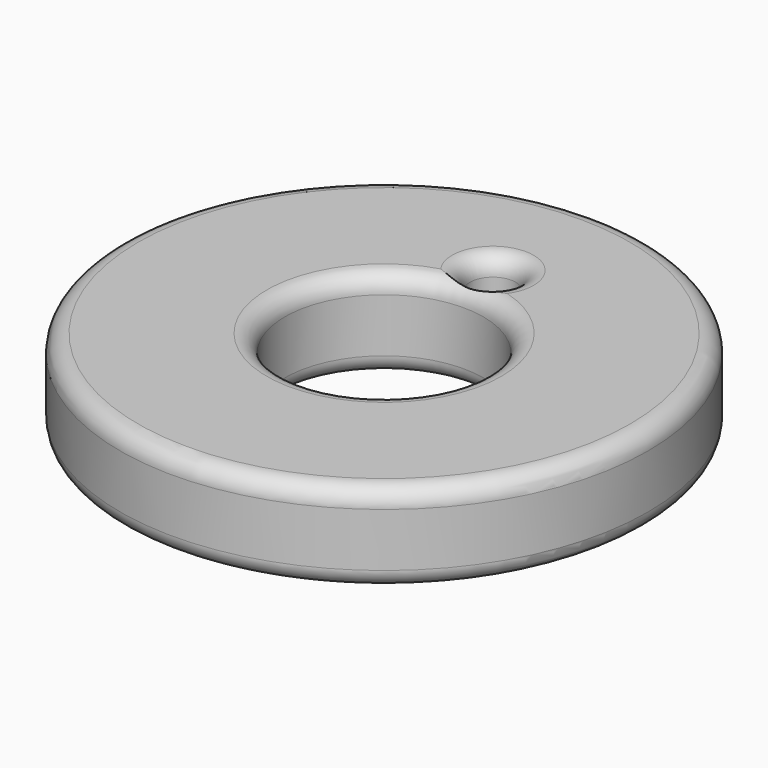
from build123d import *

# Parameters (mm, degrees)
F0_R     = 74.892271749
F0_R_2   = 28.179048931
F0_R_3   = 6.4977417518
F1_DEPTH = 25.4


# Not quite as in the source:
# - a fillet or chamfer that OpenCascade refuses, or shapes differently, is made with other operations: its cross-section is extruded or revolved along the edge and cut away or added


with BuildPart() as f1:
    # F0 (on Top) → F1 (new body)
    with BuildSketch(Plane.XY):
        Circle(F0_R)
        Circle(F0_R_2, mode=Mode.SUBTRACT)
        with Locations((0, 38.5870411992)):
            Circle(F0_R_3, mode=Mode.SUBTRACT)
    extrude(amount=F1_DEPTH)

    # F2: fillet of radius 5.08 on 7 edges, made by hand

    # F2_s1 → F2_t2 (revolve, cut)
    with BuildSketch(Plane.XZ):
        with BuildLine():
            ThreePointArc((74.892271749, 20.32), (73.4043741975, 23.9121024484), (69.812271749, 25.4))
            Line((69.812271749, 25.4), (69.812271749, 25.5016))
            Line((69.812271749, 25.5016), (74.993871749, 25.5016))
            Line((74.993871749, 25.5016), (74.993871749, 20.32))
            Line((74.993871749, 20.32), (74.892271749, 20.32))
        make_face()
    revolve(axis=Axis((0, 0, 25.4), (0, 0, 1)), mode=Mode.SUBTRACT)

    # F2_s3 → F2_t4 (revolve, cut)
    with BuildSketch(Plane.XZ):
        with BuildLine():
            ThreePointArc((28.179048931, 20.32), (29.6669464826, 23.9121024484), (33.259048931, 25.4))
            Line((33.259048931, 25.4), (33.259048931, 25.5016))
            Line((33.259048931, 25.5016), (28.077448931, 25.5016))
            Line((28.077448931, 25.5016), (28.077448931, 20.32))
            Line((28.077448931, 20.32), (28.179048931, 20.32))
        make_face()
    revolve(axis=Axis((0, 0, 25.4), (0, 0, 1)), mode=Mode.SUBTRACT)

    # F2_s5 → F2_t6 (revolve, cut)
    with BuildSketch(Plane.XZ.offset(-38.5870411992)):
        with BuildLine():
            ThreePointArc((6.4977417518, 20.32), (7.9856393033, 23.9121024484), (11.5777417518, 25.4))
            Line((11.5777417518, 25.4), (11.5777417518, 25.5016))
            Line((11.5777417518, 25.5016), (6.3961417518, 25.5016))
            Line((6.3961417518, 25.5016), (6.3961417518, 20.32))
            Line((6.3961417518, 20.32), (6.4977417518, 20.32))
        make_face()
    revolve(axis=Axis((0, 38.5870411992, 25.4), (0, 0, 1)), mode=Mode.SUBTRACT)

    # F2_s7 → F2_t8 (revolve, cut)
    with BuildSketch(Plane.XZ.offset(-38.5870411992)):
        with BuildLine():
            ThreePointArc((6.4977417518, 5.08), (7.9856393033, 1.4878975516), (11.5777417518, 0))
            Line((11.5777417518, 0), (11.5777417518, -0.1016))
            Line((11.5777417518, -0.1016), (6.3961417518, -0.1016))
            Line((6.3961417518, -0.1016), (6.3961417518, 5.08))
            Line((6.3961417518, 5.08), (6.4977417518, 5.08))
        make_face()
    revolve(axis=Axis((0, 38.5870411992, 0), (0, 0, 1)), mode=Mode.SUBTRACT)

    # F2_s9 → F2_t10 (revolve, cut)
    with BuildSketch(Plane.XZ):
        with BuildLine():
            ThreePointArc((28.179048931, 5.08), (29.6669464826, 1.4878975516), (33.259048931, 0))
            Line((33.259048931, 0), (33.259048931, -0.1016))
            Line((33.259048931, -0.1016), (28.077448931, -0.1016))
            Line((28.077448931, -0.1016), (28.077448931, 5.08))
            Line((28.077448931, 5.08), (28.179048931, 5.08))
        make_face()
    revolve(axis=Axis((0, 0, 0), (0, 0, 1)), mode=Mode.SUBTRACT)

    # F2_s11 → F2_t12 (revolve, cut)
    with BuildSketch(Plane.XZ):
        with BuildLine():
            ThreePointArc((74.892271749, 5.08), (73.4043741975, 1.4878975516), (69.812271749, 0))
            Line((69.812271749, 0), (69.812271749, -0.1016))
            Line((69.812271749, -0.1016), (74.993871749, -0.1016))
            Line((74.993871749, -0.1016), (74.993871749, 5.08))
            Line((74.993871749, 5.08), (74.892271749, 5.08))
        make_face()
    revolve(axis=Axis((0, 0, 0), (0, 0, 1)), mode=Mode.SUBTRACT)


solid = f1.part
